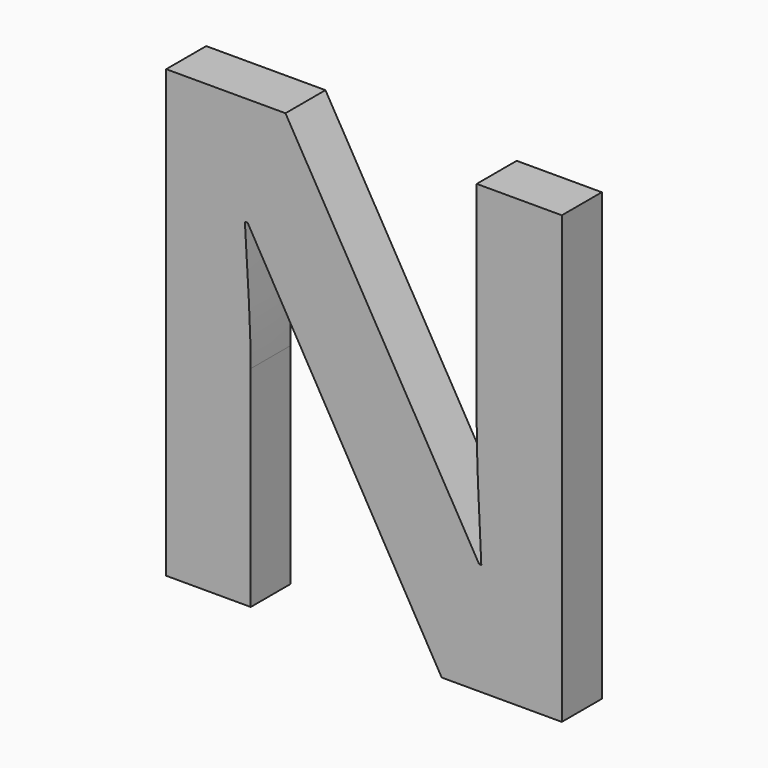
from build123d import *

# Parameters (mm, degrees)
F0_TEXT_SIZE = 62.5
F1_DEPTH     = 5


# Not quite as in the source:
# - Text() gives the source's letters only with a copy of the font that has no kerning and outlines rounded to 1/6400 em; it was checked with that copy


with BuildPart() as f1:
    # F0 (on Front) → F1 (new body)
    with BuildSketch(Plane.XZ):
        with Locations((-70.7727284726, 24.8181839512)):
            Text('N', F0_TEXT_SIZE, font='Open Sans', font_style=FontStyle.BOLD, text_align=(TextAlign.LEFT, TextAlign.BOTTOM))
    extrude(amount=F1_DEPTH)


solid = f1.part
